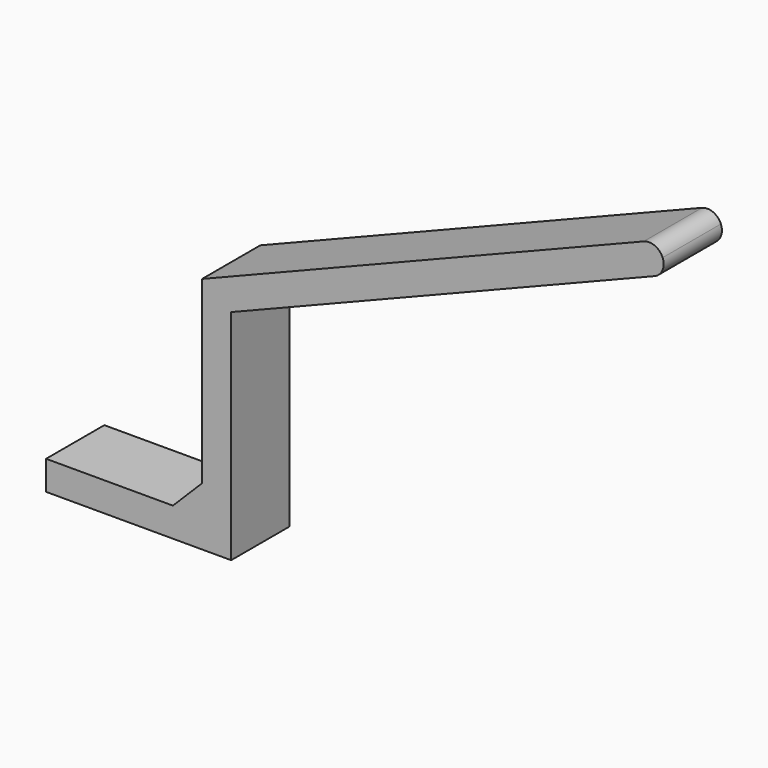
from build123d import *

# Parameters (mm, degrees)
F1_DEPTH = 5
F2_SIZE  = 2
F3_R     = 0.99999


# Not quite as in the source:
# - a fillet or chamfer is up to 0.001 mm smaller than in the source, because OpenCascade refuses the exact size


with BuildPart() as f1:
    # F0 (on Front) → F1 (new body)
    with BuildSketch(Plane.XZ):
        Polygon((-10.7482137709, -11.0476701237), (-10.7482137709, 3.9523298763), (19.2517862291, 15.9523298763), (18.5090048764, 17.8092832581), (-12.7482137709, 5.3063957992), (-12.7482137709, -9.0476701237), (-23.457470371, -9.0476701237), (-23.457470371, -11.0476701237), align=None)
    extrude(amount=F1_DEPTH)

    # F2
    f2_edges = [f1.edges().sort_by_distance(p)[0] for p in [
        (-12.748214, -2.5, -9.04767),
    ]]
    chamfer(f2_edges, length=F2_SIZE)

    # F3 (radius 1 in the source; OpenCascade refuses exactly that, so slightly less here)
    f3_edges = [f1.edges().sort_by_distance(p)[0] for p in [
        (18.509005, -2.5, 17.809283),
        (19.251786, -2.5, 15.95233),
    ]]
    fillet(f3_edges, radius=F3_R)


solid = f1.part
